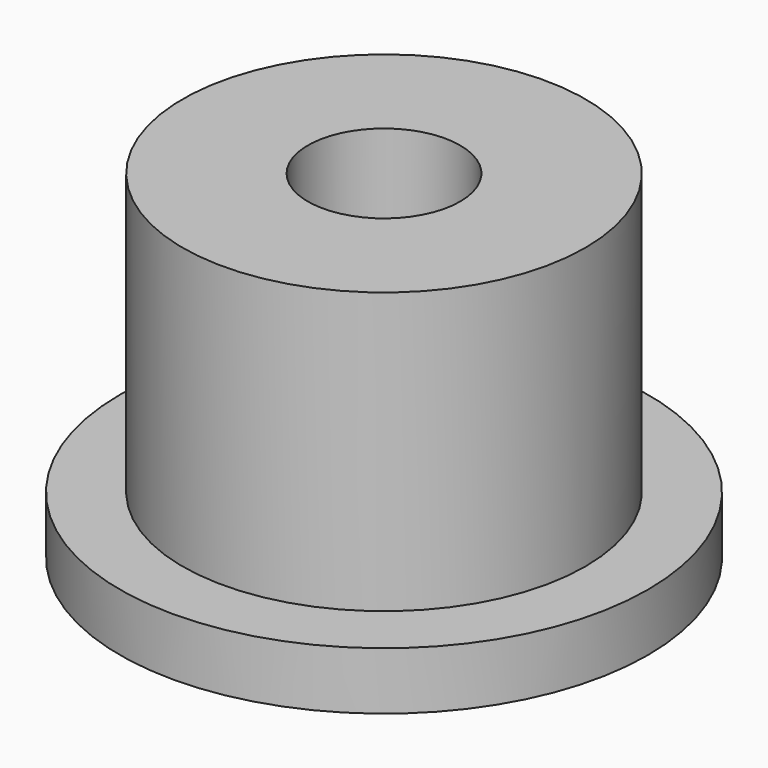
from build123d import *

# Parameters (mm, degrees)
F0_R     = 21.0753784255
F0_R_2   = 16.0753784255
F0_R_3   = 6.0753784255
F1_DEPTH = 4.6
F2_DEPTH = 27


# Not quite as in the source:
# - a feature of the source that left no trace in its solid (it failed there, or was rolled back) is left out


with BuildPart() as f1:
    # F0 (on Top) → F1 (new body)
    with BuildSketch(Plane.XY):
        with Locations((43.8603498042, 10.2871814743)):
            Circle(F0_R)
        with Locations((43.8603498042, 10.2871814743)):
            Circle(F0_R_2, mode=Mode.SUBTRACT)
        with Locations((43.8603498042, 10.2871814743)):
            Circle(F0_R_2)
        with Locations((43.8603498042, 10.2871814743)):
            Circle(F0_R_3, mode=Mode.SUBTRACT)
    extrude(amount=F1_DEPTH)

    # F0 (on Top) → F2 (join)
    with BuildSketch(Plane.XY):
        with Locations((43.8603498042, 10.2871814743)):
            Circle(F0_R_2)
        with Locations((43.8603498042, 10.2871814743)):
            Circle(F0_R_3, mode=Mode.SUBTRACT)
    extrude(amount=F2_DEPTH)


solid = f1.part
